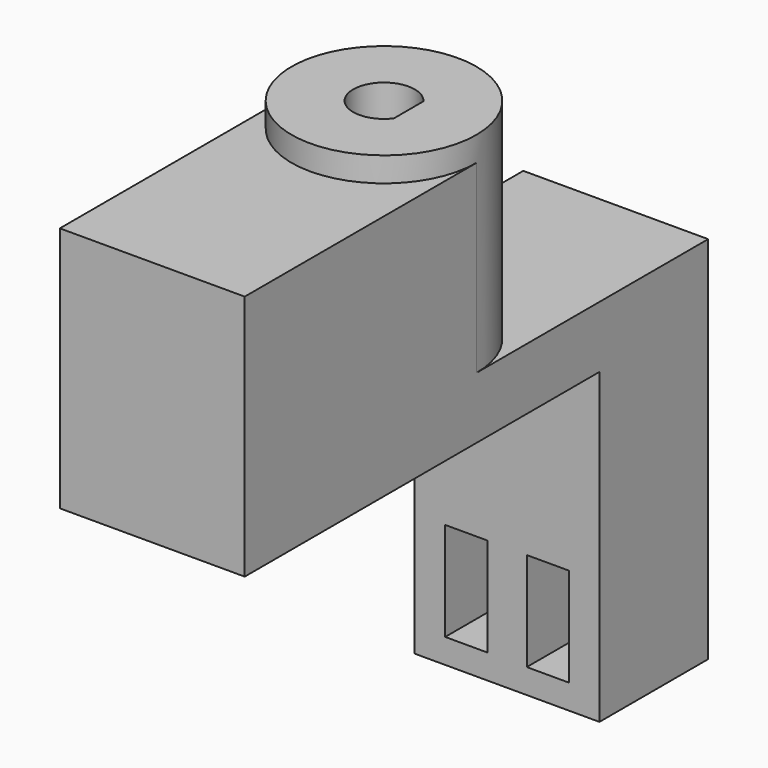
from build123d import *

# Parameters (mm, degrees)
F0_R     = 7.5
F1_DEPTH = 22
F3_DEPTH = 18
F4_W     = 15
F4_H     = 11.0249955803
F5_DEPTH = 5
F6_DEPTH = 25
F7_DEPTH = 20
F8_W     = 3.414438339
F8_H     = 8.0012119859
F9_DEPTH = 11.0259955803


with BuildPart() as f1:
    # F0 (on Top) → F1 (new body)
    with BuildSketch(Plane.XY):
        Circle(F0_R)
    extrude(amount=F1_DEPTH)

    # F2 (on face) → F3 (cut)
    with BuildSketch(Plane.XY.offset(22)):
        with BuildLine():
            Line((2, -1.5), (2, 1.5))
            ThreePointArc((2, 1.5), (-2.5, 0), (2, -1.5))
        make_face()
    extrude(amount=-F3_DEPTH, mode=Mode.SUBTRACT)

    # F4 (on face) → F5 (join)
    with BuildSketch(Plane(origin=(0, 0, 0), x_dir=(1, 0, 0), z_dir=(0, 0, -1))):
        with BuildLine():
            ThreePointArc((7.5, 0), (0, -7.5), (-7.5, 0))
            Line((-7.5, 0), (-7.5, -12.4750044197))
            Line((-7.5, -12.4750044197), (7.5, -12.4750044197))
            Line((7.5, -12.4750044197), (7.5, 0))
        make_face()
        with Locations((0, -17.9875022098)):
            Rectangle(F4_W, F4_H)
    extrude(amount=-F5_DEPTH)

    # F4 (on face) → F6 (join)
    with BuildSketch(Plane(origin=(0, 0, 0), x_dir=(1, 0, 0), z_dir=(0, 0, -1))):
        with Locations((0, -17.9875022098)):
            Rectangle(F4_W, F4_H)
    extrude(amount=F6_DEPTH)

    # F4 (on face) → F7 (join)
    with BuildSketch(Plane(origin=(0, 0, 0), x_dir=(1, 0, 0), z_dir=(0, 0, -1))):
        with BuildLine():
            Line((-7.5, 12.4750044197), (-7.5, 0))
            ThreePointArc((-7.5, 0), (0, 7.5), (7.5, 0))
            Line((7.5, 0), (7.5, 12.4750044197))
            Line((7.5, 12.4750044197), (-7.5, 12.4750044197))
        make_face()
        with Locations((0, 17.9875022098)):
            Rectangle(F4_W, F4_H)
    extrude(amount=-F7_DEPTH)

    # F8 (on face) → F9 (cut, through all)
    with BuildSketch(Plane.XZ.offset(-12.4750044197)):
        with Locations((3.3099151915, -18.999394007)):
            Rectangle(F8_W, F8_H)
        with Locations((-3.3099151915, -18.999394007)):
            Rectangle(F8_W, F8_H)
    extrude(amount=-F9_DEPTH, mode=Mode.SUBTRACT)


solid = f1.part
